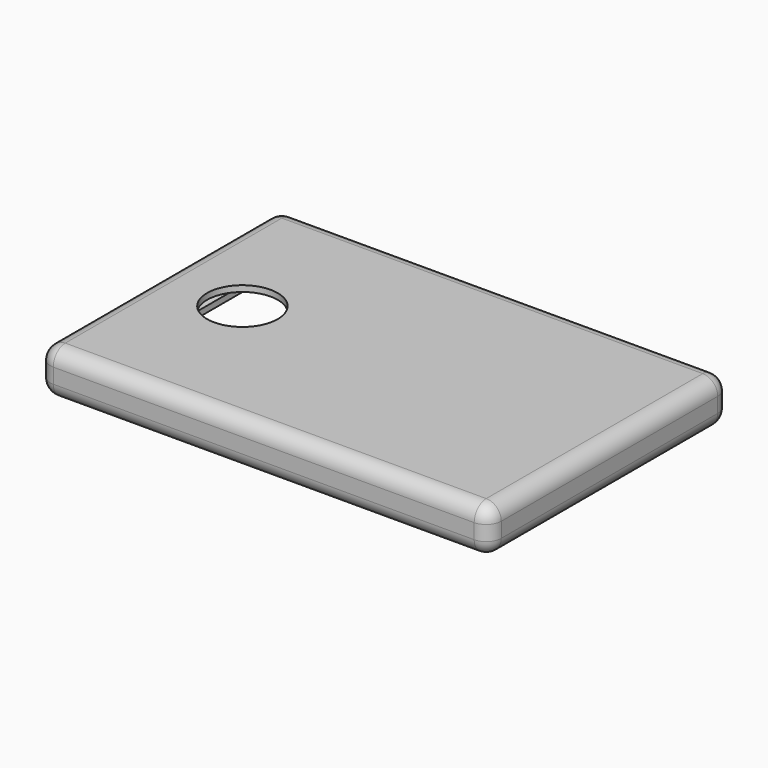
from build123d import *

# Parameters (mm, degrees)
F0_W     = 150
F0_H     = 100
F1_DEPTH = 15
F2_R     = 5
F3_T     = -2
F4_R     = 11.751583661
F5_DEPTH = 25


# Not quite as in the source:
# - a shell that OpenCascade refuses in one call is made with other operations: the cavity is built on its own and cut out


with BuildPart() as f1:
    # F0 (on Top) → F1 (new body)
    with BuildSketch(Plane.XY):
        Rectangle(F0_W, F0_H)
    extrude(amount=F1_DEPTH)

    # F2
    f2_edges = [f1.edges().sort_by_distance(p)[0] for p in [
        (0, 50, 0),
        (75, 0, 15),
        (0, 50, 15),
        (-75, 0, 15),
        (0, -50, 15),
        (-75, 50, 7.5),
        (-75, -50, 7.5),
        (-75, 0, 0),
        (75, -50, 7.5),
        (0, -50, 0),
        (75, 50, 7.5),
        (75, 0, 0),
    ]]
    fillet(f2_edges, radius=F2_R)

    # F3: a shell. OpenCascade refuses it in one call, so the cavity is built on its own and cut out:
    # the body offset inwards by the wall thickness, plus a prism from it out through each open face.
    f3_core = offset(f1.part, amount=F3_T, mode=Mode.PRIVATE)
    f3_exits = [f3_core.faces().sort_by_distance(p)[0] for p in [
        (0, 0, 2),
    ]]
    add(f3_core, mode=Mode.SUBTRACT)
    extrude(f3_exits, amount=-F3_T, mode=Mode.SUBTRACT)

    # F4 (on face) → F5 (cut)
    with BuildSketch(Plane.XY.offset(15)):
        with Locations((-47.0996387303, 0)):
            Circle(F4_R)
    extrude(amount=-F5_DEPTH, mode=Mode.SUBTRACT)


solid = f1.part
